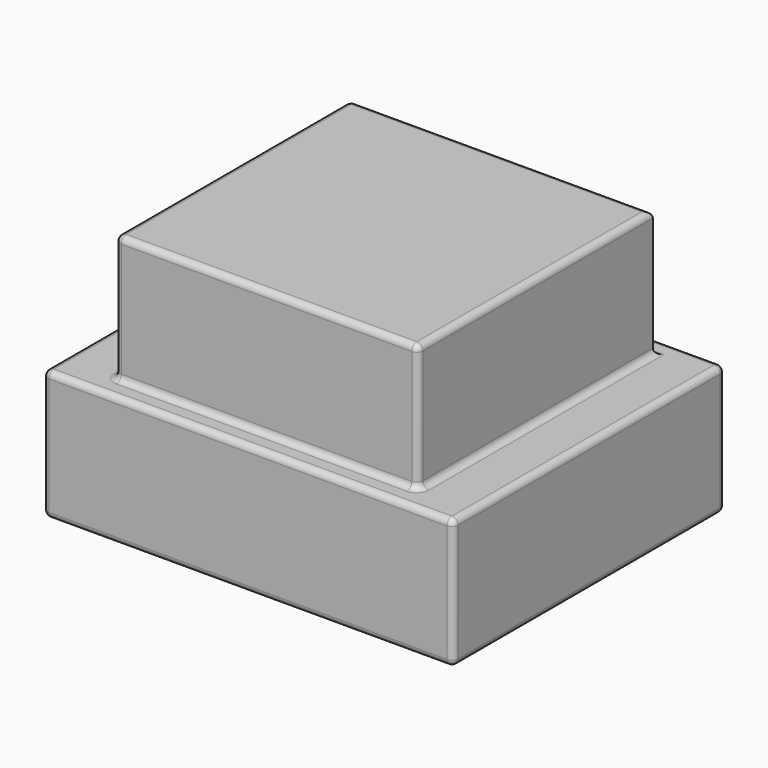
from build123d import *

# Parameters (mm, degrees)
F0_W     = 66.4
F0_H     = 55
F0_W_2   = 49
F0_H_2   = 47.5
F1_DEPTH = 21
F2_DEPTH = 41.5
F3_R     = 1


with BuildPart() as f1:
    # F0 (on Top) → F1 (new body)
    with BuildSketch(Plane.XY):
        Rectangle(F0_W, F0_H)
        Rectangle(F0_W_2, F0_H_2, mode=Mode.SUBTRACT)
    extrude(amount=F1_DEPTH)

    # F0 (on Top) → F2 (join)
    with BuildSketch(Plane.XY):
        Rectangle(F0_W_2, F0_H_2)
    extrude(amount=F2_DEPTH)

    # F3
    f3_edges = [f1.edges().sort_by_distance(p)[0] for p in [
        (0, 23.75, 41.5),
        (-24.5, 0, 41.5),
        (0, -23.75, 41.5),
        (24.5, 0, 41.5),
        (-24.5, 0, 21),
        (-24.5, -23.75, 31.25),
        (-24.5, 23.75, 31.25),
        (0, -23.75, 21),
        (24.5, -23.75, 31.25),
        (33.2, -27.5, 10.5),
        (33.2, 27.5, 10.5),
        (33.2, 0, 0),
        (33.2, 0, 21),
        (-33.2, -27.5, 10.5),
        (0, -27.5, 0),
        (0, -27.5, 21),
        (-33.2, 27.5, 10.5),
        (-33.2, 0, 0),
        (-33.2, 0, 21),
        (0, 27.5, 0),
        (0, 27.5, 21),
        (24.5, 0, 21),
        (0, 23.75, 21),
    ]]
    fillet(f3_edges, radius=F3_R)


solid = f1.part
